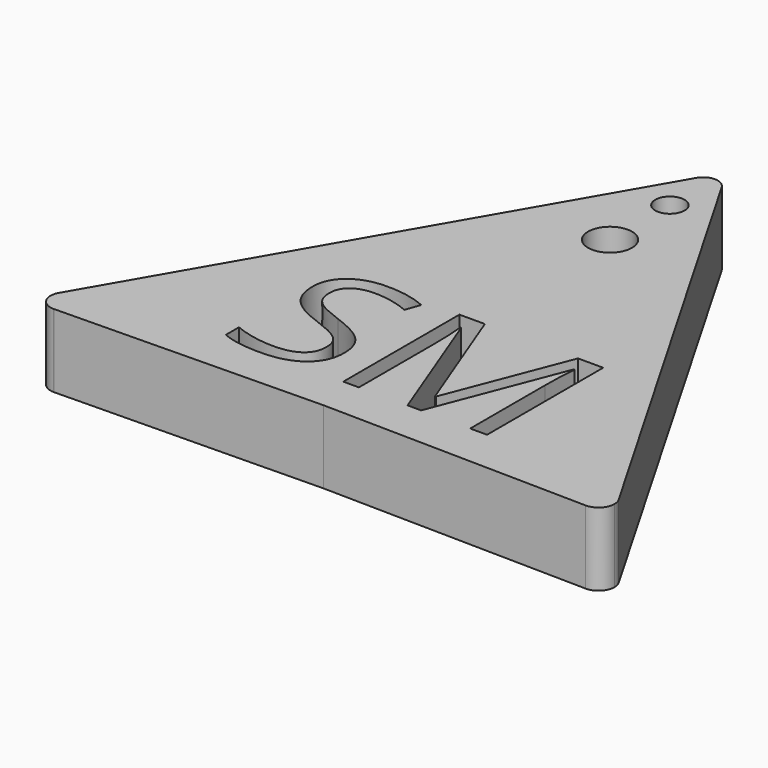
from build123d import *

# Parameters (mm, degrees)
F1_DEPTH     = 5
F2_TEXT_SIZE = 13.8888888889
F3_DEPTH     = 5.001
F4_R         = 1
F4_R_2       = 1.5
F5_DEPTH     = 5.0010001


# Not quite as in the source:
# - Text() gives the source's letters only with a copy of the font that has no kerning and outlines rounded to 1/6400 em; it was checked with that copy


with BuildPart() as f1:
    # F0 (on Top) → F1 (new body)
    with BuildSketch(Plane.XY):
        with BuildLine():
            ThreePointArc((0, 14.3205080757), (-0.8660254038, 14.8205080757), (-0.8660254038, 15.8205080757))
            Line((-0.8660254038, 15.8205080757), (-19.1129920729, -15.7841652792))
            ThreePointArc((-19.1129920729, -15.7841652792), (-18.1604730406, -15.2421357399), (-17.221798037, -15.8078015121))
            ThreePointArc((-17.221798037, -15.8078015121), (-17.1233133603, -16.0587704239), (-17.0897943042, -16.3262794875))
            ThreePointArc((-17.0897943042, -16.3262794875), (-17.4009991037, -17.086533226), (-18.1559640117, -17.4103575023))
            Line((-18.1559640117, -17.4103575023), (0, -17.1079131517))
            Line((0, -17.1079131517), (18.1559640117, -17.4103575023))
            ThreePointArc((18.1559640117, -17.4103575023), (17.2396007658, -15.7763641582), (19.1129920729, -15.7841652792))
            Line((19.1129920729, -15.7841652792), (0.8660254038, 15.8205080757))
            ThreePointArc((0.8660254038, 15.8205080757), (0.9659258263, 15.5793271208), (1, 15.3205080757))
            ThreePointArc((1, 15.3205080757), (0.7071067812, 14.6134012945), (0, 14.3205080757))
        make_face()
        with BuildLine():
            ThreePointArc((0.8660254038, 15.8205080757), (0, 16.3205080757), (-0.8660254038, 15.8205080757))
            ThreePointArc((-0.8660254038, 15.8205080757), (-0.8660254038, 14.8205080757), (0, 14.3205080757))
            ThreePointArc((0, 14.3205080757), (0.7071067812, 14.6134012945), (1, 15.3205080757))
            ThreePointArc((1, 15.3205080757), (0.9659258263, 15.5793271208), (0.8660254038, 15.8205080757))
        make_face()
        with BuildLine():
            ThreePointArc((-17.221798037, -15.8078015121), (-18.1604730406, -15.2421357399), (-19.1129920729, -15.7841652792))
            ThreePointArc((-19.1129920729, -15.7841652792), (-19.2581664682, -16.3127298075), (-19.1262474044, -16.8447574629))
            Line((-19.1262474044, -16.8447574629), (-17.221798037, -15.8078015121))
        make_face()
        with BuildLine():
            ThreePointArc((-17.0897943042, -16.3262794875), (-17.1233133603, -16.0587704239), (-17.221798037, -15.8078015121))
            Line((-17.221798037, -15.8078015121), (-19.1262474044, -16.8447574629))
            ThreePointArc((-19.1262474044, -16.8447574629), (-18.7355726443, -17.2537561408), (-18.1920814297, -17.4103575023))
            Line((-18.1920814297, -17.4103575023), (-18.1559640117, -17.4103575023))
            ThreePointArc((-18.1559640117, -17.4103575023), (-17.4009991037, -17.086533226), (-17.0897943042, -16.3262794875))
        make_face()
        with BuildLine():
            ThreePointArc((19.2582511372, -16.3262794875), (19.2213069498, -16.0456605241), (19.1129920729, -15.7841652792))
            ThreePointArc((19.1129920729, -15.7841652792), (17.2396007658, -15.7763641582), (18.1559640117, -17.4103575023))
            ThreePointArc((18.1559640117, -17.4103575023), (18.9342764592, -17.0993031044), (19.2582511372, -16.3262794875))
        make_face()
        with BuildLine():
            Line((-18.1559640117, -17.4103575023), (-18.1920814297, -17.4103575023))
            ThreePointArc((-18.1920814297, -17.4103575023), (-18.1740227207, -17.410507904), (-18.1559640117, -17.4103575023))
        make_face()
    extrude(amount=F1_DEPTH)

    # F2 (on face) → F3 (cut, through all)
    with BuildSketch(Plane.XY.offset(5)):
        with Locations((-9.853515625, -14.3205080757)):
            Text('SM', F2_TEXT_SIZE, font='Open Sans', text_align=(TextAlign.LEFT, TextAlign.BOTTOM))
    extrude(amount=-F3_DEPTH, mode=Mode.SUBTRACT)

    # F4 (on face) → F5 (cut, through all)
    with BuildSketch(Plane.XY.offset(5)):
        with Locations((0, 12.4804219231)):
            Circle(F4_R)
        with Locations((0, 7.3673807555)):
            Circle(F4_R_2)
    extrude(amount=-F5_DEPTH, mode=Mode.SUBTRACT)


solid = f1.part
